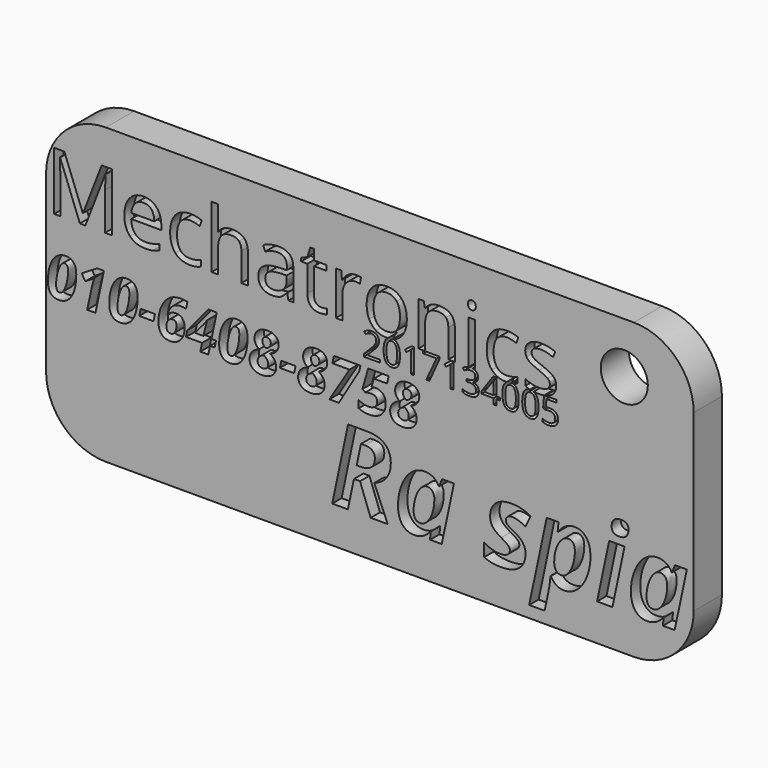
from build123d import *

# Parameters (mm, degrees)
F0_W           = 55
F0_H           = 25
F1_DEPTH       = 3
F2_TEXT_SIZE   = 4.7299554753
F2_TEXT_SIZE_2 = 8.9130162028
F3_DEPTH       = 1
F4_R           = 5.08
F5_R           = 5.08
F6_R           = 5.08
F7_R           = 5.08
F8_R           = 2
F9_DEPTH       = 3


# Not quite as in the source:
# - Text() gives the source's letters only with a copy of the font that has no kerning and outlines rounded to 1/6400 em; it was checked with that copy


with BuildPart() as f1:
    # F0 (on Front) → F1 (new body)
    with BuildSketch(Plane.XZ):
        with Locations((3.4295588825, -2.7567299395)):
            Rectangle(F0_W, F0_H)
    extrude(amount=F1_DEPTH)

    # F2 (on face) → F3 (cut)
    with BuildSketch(Plane.XZ.offset(3)):
        with Locations((-24.0704411175, -4.4084611423)):
            Text('010-6408-8758', F2_TEXT_SIZE, font='Open Sans', font_style=FontStyle.BOLDITALIC, text_align=(TextAlign.LEFT, TextAlign.BOTTOM))
        with Locations((0, -12.1290959666)):
            Text('Ra spia', F2_TEXT_SIZE_2, font='Open Sans', font_style=FontStyle.BOLDITALIC, text_align=(TextAlign.LEFT, TextAlign.BOTTOM))
        with BuildLine():
            Line((-22.8788005036, 6.2329982247), (-21.1996705477, 1.8455941463))
            Line((-21.1996705477, 1.8455941463), (-20.7360140179, 1.8455941463))
            Line((-20.7360140179, 1.8455941463), (-19.0428010365, 6.2264983668))
            Line((-19.0428010365, 6.2264983668), (-19.0157182953, 6.2264983668))
            add(Edge.make_bspline(
                [(-19.0633839198, 5.0348577529), (-19.0633839198, 5.5830124353), (-19.0157182953, 6.2264983668)],
                knots=[0, 0, 0, 1, 1, 1], degree=2))
            Line((-19.0633839198, 5.0348577529), (-19.0633839198, 1.8455941463))
            Line((-19.0633839198, 1.8455941463), (-18.4881464962, 1.8455941463))
            Line((-18.4881464962, 1.8455941463), (-18.4881464962, 6.7952359326))
            Line((-18.4881464962, 6.7952359326), (-19.3482943575, 6.7952359326))
            Line((-19.3482943575, 6.7952359326), (-20.9288431354, 2.7122418655))
            Line((-20.9288431354, 2.7122418655), (-20.9559258766, 2.7122418655))
            Line((-20.9559258766, 2.7122418655), (-22.5234749387, 6.7952359326))
            Line((-22.5234749387, 6.7952359326), (-23.3901226579, 6.7952359326))
            Line((-23.3901226579, 6.7952359326), (-23.3901226579, 1.8455941463))
            Line((-23.3901226579, 1.8455941463), (-22.8582176203, 1.8455941463))
            Line((-22.8582176203, 1.8455941463), (-22.8582176203, 4.9936919863))
            add(Edge.make_bspline(
                [(-22.9058832448, 6.2329982247), (-22.8582176203, 5.7119262836), (-22.8582176203, 4.9936919863)],
                knots=[0, 0, 0, 1, 1, 1], degree=2))
            Line((-22.9058832448, 6.2329982247), (-22.8788005036, 6.2329982247))
        make_face()
        with BuildLine():
            add(Edge.make_bspline(
                [(-15.6477085965, 1.7773456384), (-16.4699406201, 1.7773456384), (-16.9460552109, 2.2789180059)],
                knots=[0, 0, 0, 1, 1, 1], degree=2))
            add(Edge.make_bspline(
                [(-15.0063892843, 1.8336777401), (-15.2718001483, 1.7773456384), (-15.6477085965, 1.7773456384)],
                knots=[0, 0, 0, 1, 1, 1], degree=2))
            add(Edge.make_bspline(
                [(-14.4430682669, 2.0178403805), (-14.7409784203, 1.8900098419), (-15.0063892843, 1.8336777401)],
                knots=[0, 0, 0, 1, 1, 1], degree=2))
            Line((-14.4430682669, 2.0178403805), (-14.4430682669, 2.519412748))
            add(Edge.make_bspline(
                [(-15.6271257132, 2.269168219), (-15.0280554773, 2.269168219), (-14.4430682669, 2.519412748)],
                knots=[0, 0, 0, 1, 1, 1], degree=2))
            add(Edge.make_bspline(
                [(-16.5089397675, 2.6077024844), (-16.1958632789, 2.269168219), (-15.6271257132, 2.269168219)],
                knots=[0, 0, 0, 1, 1, 1], degree=2))
            add(Edge.make_bspline(
                [(-16.8393492104, 3.599472468), (-16.8220162561, 2.9462367497), (-16.5089397675, 2.6077024844)],
                knots=[0, 0, 0, 1, 1, 1], degree=2))
            Line((-16.8393492104, 3.599472468), (-14.2838217485, 3.599472468))
            Line((-14.2838217485, 3.599472468), (-14.2838217485, 3.9547980329))
            add(Edge.make_bspline(
                [(-14.6900628668, 5.1653965656), (-14.2838217485, 4.7066149293), (-14.2838217485, 3.9547980329)],
                knots=[0, 0, 0, 1, 1, 1], degree=2))
            add(Edge.make_bspline(
                [(-15.7928720895, 5.624178202), (-15.0963039852, 5.624178202), (-14.6900628668, 5.1653965656)],
                knots=[0, 0, 0, 1, 1, 1], degree=2))
            add(Edge.make_bspline(
                [(-16.9801794648, 5.0960647481), (-16.538189128, 5.624178202), (-15.7928720895, 5.624178202)],
                knots=[0, 0, 0, 1, 1, 1], degree=2))
            add(Edge.make_bspline(
                [(-17.4221698016, 3.6698875952), (-17.4221698016, 4.5679512942), (-16.9801794648, 5.0960647481)],
                knots=[0, 0, 0, 1, 1, 1], degree=2))
            add(Edge.make_bspline(
                [(-16.9460552109, 2.2789180059), (-17.4221698016, 2.7804903734), (-17.4221698016, 3.6698875952)],
                knots=[0, 0, 0, 1, 1, 1], degree=2))
        make_face()
        with BuildLine():
            add(Edge.make_bspline(
                [(-15.8004552571, 5.1529385047), (-16.2467788324, 5.1529385047), (-16.5127313513, 4.8620698639)],
                knots=[0, 0, 0, 1, 1, 1], degree=2))
            add(Edge.make_bspline(
                [(-15.1228450716, 4.8701946863), (-15.3595482299, 5.1529385047), (-15.8004552571, 5.1529385047)],
                knots=[0, 0, 0, 1, 1, 1], degree=2))
            add(Edge.make_bspline(
                [(-14.8861419133, 4.0566291399), (-14.8861419133, 4.5874508679), (-15.1228450716, 4.8701946863)],
                knots=[0, 0, 0, 1, 1, 1], degree=2))
            Line((-14.8861419133, 4.0566291399), (-16.8263494947, 4.0566291399))
            add(Edge.make_bspline(
                [(-16.5127313513, 4.8620698639), (-16.7786838701, 4.5712012232), (-16.8263494947, 4.0566291399)],
                knots=[0, 0, 0, 1, 1, 1], degree=2))
        make_face(mode=Mode.SUBTRACT)
        with BuildLine():
            add(Edge.make_bspline(
                [(-11.8420417996, 1.7773456384), (-12.6480241785, 1.7773456384), (-13.0900145153, 2.2735014576)],
                knots=[0, 0, 0, 1, 1, 1], degree=2))
            add(Edge.make_bspline(
                [(-10.9049789532, 1.9712580656), (-11.2765541628, 1.7773456384), (-11.8420417996, 1.7773456384)],
                knots=[0, 0, 0, 1, 1, 1], degree=2))
            Line((-10.9049789532, 1.9712580656), (-10.9049789532, 2.4684971945))
            add(Edge.make_bspline(
                [(-11.8561248251, 2.269168219), (-11.3924682953, 2.269168219), (-10.9049789532, 2.4684971945)],
                knots=[0, 0, 0, 1, 1, 1], degree=2))
            add(Edge.make_bspline(
                [(-12.6734819552, 2.6347852256), (-12.3977796496, 2.269168219), (-11.8561248251, 2.269168219)],
                knots=[0, 0, 0, 1, 1, 1], degree=2))
            add(Edge.make_bspline(
                [(-12.9491842609, 3.6839706206), (-12.9491842609, 3.0004022321), (-12.6734819552, 2.6347852256)],
                knots=[0, 0, 0, 1, 1, 1], degree=2))
            add(Edge.make_bspline(
                [(-11.8182089873, 5.1258557635), (-12.9491842609, 5.1258557635), (-12.9491842609, 3.6839706206)],
                knots=[0, 0, 0, 1, 1, 1], degree=2))
            add(Edge.make_bspline(
                [(-11.4293008233, 5.0771068293), (-11.6492126821, 5.1258557635), (-11.8182089873, 5.1258557635)],
                knots=[0, 0, 0, 1, 1, 1], degree=2))
            add(Edge.make_bspline(
                [(-11.023059705, 4.9536095293), (-11.2093889646, 5.028357895), (-11.4293008233, 5.0771068293)],
                knots=[0, 0, 0, 1, 1, 1], degree=2))
            Line((-11.023059705, 4.9536095293), (-10.8508134708, 5.4302657748))
            add(Edge.make_bspline(
                [(-11.2700543049, 5.5662211358), (-11.0024768216, 5.5082640696), (-10.8508134708, 5.4302657748)],
                knots=[0, 0, 0, 1, 1, 1], degree=2))
            add(Edge.make_bspline(
                [(-11.8052092716, 5.624178202), (-11.5376317882, 5.624178202), (-11.2700543049, 5.5662211358)],
                knots=[0, 0, 0, 1, 1, 1], degree=2))
            add(Edge.make_bspline(
                [(-13.0829730025, 5.1161059766), (-12.633941153, 5.624178202), (-11.8052092716, 5.624178202)],
                knots=[0, 0, 0, 1, 1, 1], degree=2))
            add(Edge.make_bspline(
                [(-13.5320048521, 3.6774707627), (-13.5320048521, 4.6080337512), (-13.0829730025, 5.1161059766)],
                knots=[0, 0, 0, 1, 1, 1], degree=2))
            add(Edge.make_bspline(
                [(-13.0900145153, 2.2735014576), (-13.5320048521, 2.7696572769), (-13.5320048521, 3.6774707627)],
                knots=[0, 0, 0, 1, 1, 1], degree=2))
        make_face()
        with BuildLine():
            Line((-7.4849703913, 4.2462083285), (-7.4849703913, 1.8455941463))
            Line((-7.4849703913, 1.8455941463), (-6.9227326835, 1.8455941463))
            Line((-6.9227326835, 1.8455941463), (-6.9227326835, 4.2657079022))
            add(Edge.make_bspline(
                [(-7.2634335681, 5.2932271042), (-6.9227326835, 4.969859174), (-6.9227326835, 4.2657079022)],
                knots=[0, 0, 0, 1, 1, 1], degree=2))
            add(Edge.make_bspline(
                [(-8.2844529123, 5.6165950345), (-7.6041344527, 5.6165950345), (-7.2634335681, 5.2932271042)],
                knots=[0, 0, 0, 1, 1, 1], degree=2))
            add(Edge.make_bspline(
                [(-8.9831876359, 5.4627650643), (-8.6766110052, 5.6165950345), (-8.2844529123, 5.6165950345)],
                knots=[0, 0, 0, 1, 1, 1], degree=2))
            add(Edge.make_bspline(
                [(-9.4555106429, 5.0413576108), (-9.2897642666, 5.3089350941), (-8.9831876359, 5.4627650643)],
                knots=[0, 0, 0, 1, 1, 1], degree=2))
            Line((-9.4555106429, 5.0413576108), (-9.489093242, 5.0413576108))
            add(Edge.make_bspline(
                [(-9.4620105008, 5.519097166), (-9.4620105008, 5.2309367994), (-9.489093242, 5.0413576108)],
                knots=[0, 0, 0, 1, 1, 1], degree=2))
            Line((-9.4620105008, 5.519097166), (-9.4620105008, 7.1137289694))
            Line((-9.4620105008, 7.1137289694), (-10.0242482086, 7.1137289694))
            Line((-10.0242482086, 7.1137289694), (-10.0242482086, 1.8455941463))
            Line((-10.0242482086, 1.8455941463), (-9.4620105008, 1.8455941463))
            Line((-9.4620105008, 1.8455941463), (-9.4620105008, 3.7858017276))
            add(Edge.make_bspline(
                [(-9.192808053, 4.82794561), (-9.4620105008, 4.5094525732), (-9.4620105008, 3.7858017276)],
                knots=[0, 0, 0, 1, 1, 1], degree=2))
            add(Edge.make_bspline(
                [(-8.3386183948, 5.1464386468), (-8.9236056052, 5.1464386468), (-9.192808053, 4.82794561)],
                knots=[0, 0, 0, 1, 1, 1], degree=2))
            add(Edge.make_bspline(
                [(-7.6913408795, 4.9227352043), (-7.8977113676, 5.1464386468), (-8.3386183948, 5.1464386468)],
                knots=[0, 0, 0, 1, 1, 1], degree=2))
            add(Edge.make_bspline(
                [(-7.4849703913, 4.2462083285), (-7.4849703913, 4.6990317618), (-7.6913408795, 4.9227352043)],
                knots=[0, 0, 0, 1, 1, 1], degree=2))
        make_face()
        with BuildLine():
            Line((-3.5991386804, 2.374249255), (-3.4875577865, 1.8455941463))
            Line((-3.4875577865, 1.8455941463), (-3.0704835717, 1.8455941463))
            Line((-3.0704835717, 1.8455941463), (-3.0704835717, 4.3783721056))
            add(Edge.make_bspline(
                [(-3.390601573, 5.3224764647), (-3.0704835717, 5.028357895), (-3.0704835717, 4.3783721056)],
                knots=[0, 0, 0, 1, 1, 1], degree=2))
            add(Edge.make_bspline(
                [(-4.3737050794, 5.6165950345), (-3.7107195742, 5.6165950345), (-3.390601573, 5.3224764647)],
                knots=[0, 0, 0, 1, 1, 1], degree=2))
            add(Edge.make_bspline(
                [(-5.0296490719, 5.5320968818), (-4.7030312127, 5.6165950345), (-4.3737050794, 5.6165950345)],
                knots=[0, 0, 0, 1, 1, 1], degree=2))
            add(Edge.make_bspline(
                [(-5.6303442723, 5.2991853073), (-5.3562669311, 5.4475987292), (-5.0296490719, 5.5320968818)],
                knots=[0, 0, 0, 1, 1, 1], degree=2))
            Line((-5.6303442723, 5.2991853073), (-5.4570147284, 4.8691113766))
            add(Edge.make_bspline(
                [(-4.4083709882, 5.1529385047), (-4.872027518, 5.1529385047), (-5.4570147284, 4.8691113766)],
                knots=[0, 0, 0, 1, 1, 1], degree=2))
            add(Edge.make_bspline(
                [(-3.807134133, 4.9449430521), (-3.9945467023, 5.1529385047), (-4.4083709882, 5.1529385047)],
                knots=[0, 0, 0, 1, 1, 1], degree=2))
            add(Edge.make_bspline(
                [(-3.6197215637, 4.3003738109), (-3.6197215637, 4.7369475995), (-3.807134133, 4.9449430521)],
                knots=[0, 0, 0, 1, 1, 1], degree=2))
            Line((-3.6197215637, 4.3003738109), (-3.6197215637, 4.0696288557))
            Line((-3.6197215637, 4.0696288557), (-4.2491244698, 4.0490459724))
            add(Edge.make_bspline(
                [(-6.0463351775, 2.8714883839), (-6.0463351775, 3.9948804899), (-4.2491244698, 4.0490459724)],
                knots=[0, 0, 0, 1, 1, 1], degree=2))
            add(Edge.make_bspline(
                [(-5.7332586889, 2.0622560761), (-6.0463351775, 2.3471665138), (-6.0463351775, 2.8714883839)],
                knots=[0, 0, 0, 1, 1, 1], degree=2))
            add(Edge.make_bspline(
                [(-4.868777589, 1.7773456384), (-5.4201822004, 1.7773456384), (-5.7332586889, 2.0622560761)],
                knots=[0, 0, 0, 1, 1, 1], degree=2))
            add(Edge.make_bspline(
                [(-4.1792509974, 1.9013845932), (-4.4549533031, 1.7773456384), (-4.868777589, 1.7773456384)],
                knots=[0, 0, 0, 1, 1, 1], degree=2))
            add(Edge.make_bspline(
                [(-3.6262214216, 2.374249255), (-3.9035486918, 2.025423548), (-4.1792509974, 1.9013845932)],
                knots=[0, 0, 0, 1, 1, 1], degree=2))
            Line((-3.6262214216, 2.374249255), (-3.5991386804, 2.374249255))
        make_face()
        with BuildLine():
            add(Edge.make_bspline(
                [(-4.7571966952, 2.2420854778), (-4.2317915154, 2.2420854778), (-3.9322563975, 2.5297041896)],
                knots=[0, 0, 0, 1, 1, 1], degree=2))
            add(Edge.make_bspline(
                [(-5.2728520881, 2.4007903414), (-5.0886894478, 2.2420854778), (-4.7571966952, 2.2420854778)],
                knots=[0, 0, 0, 1, 1, 1], degree=2))
            add(Edge.make_bspline(
                [(-5.4570147284, 2.864988526), (-5.4570147284, 2.559495205), (-5.2728520881, 2.4007903414)],
                knots=[0, 0, 0, 1, 1, 1], degree=2))
            add(Edge.make_bspline(
                [(-5.1612711942, 3.4386009851), (-5.4570147284, 3.25389669), (-5.4570147284, 2.864988526)],
                knots=[0, 0, 0, 1, 1, 1], degree=2))
            add(Edge.make_bspline(
                [(-4.1949589873, 3.6471380926), (-4.8655276601, 3.6233052803), (-5.1612711942, 3.4386009851)],
                knots=[0, 0, 0, 1, 1, 1], degree=2))
            Line((-4.1949589873, 3.6471380926), (-3.6327212795, 3.6698875952))
            Line((-3.6327212795, 3.6698875952), (-3.6327212795, 3.3351449137))
            add(Edge.make_bspline(
                [(-3.9322563975, 2.5297041896), (-3.6327212795, 2.8173229014), (-3.6327212795, 3.3351449137)],
                knots=[0, 0, 0, 1, 1, 1], degree=2))
        make_face(mode=Mode.SUBTRACT)
        with BuildLine():
            add(Edge.make_bspline(
                [(-0.7153683948, 2.2420854778), (-0.5658716632, 2.2420854778), (-0.4272080281, 2.2637516708)],
                knots=[0, 0, 0, 1, 1, 1], degree=2))
            add(Edge.make_bspline(
                [(-1.1519421833, 2.4213732247), (-0.9926956649, 2.2420854778), (-0.7153683948, 2.2420854778)],
                knots=[0, 0, 0, 1, 1, 1], degree=2))
            add(Edge.make_bspline(
                [(-1.3111887017, 2.9354036532), (-1.3111887017, 2.6006609716), (-1.1519421833, 2.4213732247)],
                knots=[0, 0, 0, 1, 1, 1], degree=2))
            Line((-1.3111887017, 2.9354036532), (-1.3111887017, 5.1193559056))
            Line((-1.3111887017, 5.1193559056), (-0.2343789106, 5.1193559056))
            Line((-0.2343789106, 5.1193559056), (-0.2343789106, 5.5559296941))
            Line((-0.2343789106, 5.5559296941), (-1.3111887017, 5.5559296941))
            Line((-1.3111887017, 5.5559296941), (-1.3111887017, 6.4160775554))
            Line((-1.3111887017, 6.4160775554), (-1.6361815964, 6.4160775554))
            Line((-1.6361815964, 6.4160775554), (-1.8723430999, 5.624178202))
            Line((-1.8723430999, 5.624178202), (-2.4042481375, 5.3901833178))
            Line((-2.4042481375, 5.3901833178), (-2.4042481375, 5.1193559056))
            Line((-2.4042481375, 5.1193559056), (-1.8723430999, 5.1193559056))
            Line((-1.8723430999, 5.1193559056), (-1.8723430999, 2.9115708409))
            add(Edge.make_bspline(
                [(-0.7966166184, 1.7773456384), (-1.8723430999, 1.7773456384), (-1.8723430999, 2.9115708409)],
                knots=[0, 0, 0, 1, 1, 1], degree=2))
            add(Edge.make_bspline(
                [(-0.4759569623, 1.8065949989), (-0.6536197448, 1.7773456384), (-0.7966166184, 1.7773456384)],
                knots=[0, 0, 0, 1, 1, 1], degree=2))
            add(Edge.make_bspline(
                [(-0.2072961694, 1.8791767454), (-0.2982941799, 1.8358443594), (-0.4759569623, 1.8065949989)],
                knots=[0, 0, 0, 1, 1, 1], degree=2))
            Line((-0.2072961694, 1.8791767454), (-0.2072961694, 2.3092506761))
            add(Edge.make_bspline(
                [(-0.4272080281, 2.2637516708), (-0.2885443931, 2.2854178638), (-0.2072961694, 2.3092506761)],
                knots=[0, 0, 0, 1, 1, 1], degree=2))
        make_face()
        with BuildLine():
            add(Edge.make_bspline(
                [(2.2269006119, 5.624178202), (2.4738952119, 5.624178202), (2.6699742584, 5.5830124353)],
                knots=[0, 0, 0, 1, 1, 1], degree=2))
            add(Edge.make_bspline(
                [(1.5866646094, 5.4275575007), (1.8780749049, 5.624178202), (2.2269006119, 5.624178202)],
                knots=[0, 0, 0, 1, 1, 1], degree=2))
            add(Edge.make_bspline(
                [(1.0894254805, 4.8691113766), (1.2952543138, 5.2309367994), (1.5866646094, 5.4275575007)],
                knots=[0, 0, 0, 1, 1, 1], degree=2))
            Line((1.0894254805, 4.8691113766), (1.0623427393, 4.8691113766))
            Line((1.0623427393, 4.8691113766), (0.9973441603, 5.5559296941))
            Line((0.9973441603, 5.5559296941), (0.5336876305, 5.5559296941))
            Line((0.5336876305, 5.5559296941), (0.5336876305, 1.8455941463))
            Line((0.5336876305, 1.8455941463), (1.0959253384, 1.8455941463))
            Line((1.0959253384, 1.8455941463), (1.0959253384, 3.8367172811))
            add(Edge.make_bspline(
                [(1.4155016848, 4.7472390411), (1.0959253384, 4.3816220346), (1.0959253384, 3.8367172811)],
                knots=[0, 0, 0, 1, 1, 1], degree=2))
            add(Edge.make_bspline(
                [(2.1857348453, 5.1128560477), (1.7350780313, 5.1128560477), (1.4155016848, 4.7472390411)],
                knots=[0, 0, 0, 1, 1, 1], degree=2))
            add(Edge.make_bspline(
                [(2.5919759636, 5.0619404942), (2.362314318, 5.1128560477), (2.1857348453, 5.1128560477)],
                knots=[0, 0, 0, 1, 1, 1], degree=2))
            Line((2.5919759636, 5.0619404942), (2.6699742584, 5.5830124353))
        make_face()
        with BuildLine():
            add(Edge.make_bspline(
                [(6.5666390658, 3.704553504), (6.5666390658, 2.7967400181), (6.1100240488, 2.2870428283)],
                knots=[0, 0, 0, 1, 1, 1], degree=2))
            add(Edge.make_bspline(
                [(6.1078574295, 5.1058145349), (6.5666390658, 4.5874508679), (6.5666390658, 3.704553504)],
                knots=[0, 0, 0, 1, 1, 1], degree=2))
            add(Edge.make_bspline(
                [(4.8712594651, 5.624178202), (5.6490757931, 5.624178202), (6.1078574295, 5.1058145349)],
                knots=[0, 0, 0, 1, 1, 1], degree=2))
            add(Edge.make_bspline(
                [(3.6113703433, 5.1177309411), (4.0652770863, 5.624178202), (4.8712594651, 5.624178202)],
                knots=[0, 0, 0, 1, 1, 1], degree=2))
            add(Edge.make_bspline(
                [(3.1574636004, 3.704553504), (3.1574636004, 4.6112836802), (3.6113703433, 5.1177309411)],
                knots=[0, 0, 0, 1, 1, 1], degree=2))
            add(Edge.make_bspline(
                [(3.3676256723, 2.6819091953), (3.1574636004, 3.1184829839), (3.1574636004, 3.704553504)],
                knots=[0, 0, 0, 1, 1, 1], degree=2))
            add(Edge.make_bspline(
                [(3.9634459793, 2.0113405226), (3.5777877442, 2.2453354068), (3.3676256723, 2.6819091953)],
                knots=[0, 0, 0, 1, 1, 1], degree=2))
            add(Edge.make_bspline(
                [(4.8474266529, 1.7773456384), (4.3491042143, 1.7773456384), (3.9634459793, 2.0113405226)],
                knots=[0, 0, 0, 1, 1, 1], degree=2))
            add(Edge.make_bspline(
                [(4.955877792, 1.7797225946), (4.9024668541, 1.7773456384), (4.8474266529, 1.7773456384)],
                knots=[0.9317104162, 0.9317104162, 0.9317104162, 1, 1, 1], degree=2))
            add(Edge.make_bspline(
                [(4.955877792, 1.7797225946), (5.0945894967, 1.8607604798), (5.2879334835, 1.8607604798)],
                knots=[0.4479110722, 0.4479110722, 0.4479110722, 1, 1, 1], degree=2))
            add(Edge.make_bspline(
                [(5.2879334835, 1.8607604798), (5.3518272745, 1.8607604798), (5.409976095, 1.8510758715)],
                knots=[0, 0, 0, 0.1868611686, 0.1868611686, 0.1868611686], degree=2))
            add(Edge.make_bspline(
                [(6.1100240488, 2.2870428283), (5.8270758606, 1.9712014937), (5.409976095, 1.8510758715)],
                knots=[0, 0, 0, 0.6196646574, 0.6196646574, 0.6196646574], degree=2))
        make_face()
        with BuildLine():
            add(Edge.make_bspline(
                [(3.7402841916, 3.704553504), (3.7402841916, 2.9928190646), (4.0246529744, 2.6207022001)],
                knots=[0, 0, 0, 1, 1, 1], degree=2))
            add(Edge.make_bspline(
                [(4.0214030455, 4.7840715692), (3.7402841916, 4.4217044916), (3.7402841916, 3.704553504)],
                knots=[0, 0, 0, 1, 1, 1], degree=2))
            add(Edge.make_bspline(
                [(4.8539265107, 5.1464386468), (4.3025218994, 5.1464386468), (4.0214030455, 4.7840715692)],
                knots=[0, 0, 0, 1, 1, 1], degree=2))
            add(Edge.make_bspline(
                [(5.698908037, 4.7791966758), (5.4129142896, 5.1464386468), (4.8539265107, 5.1464386468)],
                knots=[0, 0, 0, 1, 1, 1], degree=2))
            add(Edge.make_bspline(
                [(5.9849017843, 3.704553504), (5.9849017843, 4.4119547048), (5.698908037, 4.7791966758)],
                knots=[0, 0, 0, 1, 1, 1], degree=2))
            add(Edge.make_bspline(
                [(5.698908037, 2.6190772357), (5.9849017843, 2.9895691356), (5.9849017843, 3.704553504)],
                knots=[0, 0, 0, 1, 1, 1], degree=2))
            add(Edge.make_bspline(
                [(4.8604263686, 2.2485853357), (5.4129142896, 2.2485853357), (5.698908037, 2.6190772357)],
                knots=[0, 0, 0, 1, 1, 1], degree=2))
            add(Edge.make_bspline(
                [(4.0246529744, 2.6207022001), (4.3090217573, 2.2485853357), (4.8604263686, 2.2485853357)],
                knots=[0, 0, 0, 1, 1, 1], degree=2))
        make_face(mode=Mode.SUBTRACT)
        with BuildLine():
            add(Edge.make_bspline(
                [(5.409976095, 1.8510758715), (5.6630145634, 1.8089326533), (5.8072655083, 1.5834004116)],
                knots=[0.1868611686, 0.1868611686, 0.1868611686, 1, 1, 1], degree=2))
            add(Edge.make_bspline(
                [(5.409976095, 1.8510758715), (5.1999363399, 1.7905839741), (4.955877792, 1.7797225946)],
                knots=[0.6196646574, 0.6196646574, 0.6196646574, 0.9317104162, 0.9317104162, 0.9317104162], degree=2))
            add(Edge.make_bspline(
                [(4.7667631152, 1.5948900582), (4.8433406531, 1.7139763638), (4.955877792, 1.7797225946)],
                knots=[0, 0, 0, 0.4479110722, 0.4479110722, 0.4479110722], degree=2))
            add(Edge.make_bspline(
                [(4.5957971743, 0.7807337024), (4.5957971743, 1.3290196366), (4.7667631152, 1.5948900582)],
                knots=[0, 0, 0, 1, 1, 1], degree=2))
            add(Edge.make_bspline(
                [(4.7725079385, -0.0260692796), (4.5957971743, 0.2489928593), (4.5957971743, 0.7807337024)],
                knots=[0, 0, 0, 1, 1, 1], degree=2))
            add(Edge.make_bspline(
                [(5.2879334835, -0.3011314184), (4.9492187027, -0.3011314184), (4.7725079385, -0.0260692796)],
                knots=[0, 0, 0, 1, 1, 1], degree=2))
            add(Edge.make_bspline(
                [(5.8130103316, -0.0325034816), (5.6413550119, -0.3011314184), (5.2879334835, -0.3011314184)],
                knots=[0, 0, 0, 1, 1, 1], degree=2))
            add(Edge.make_bspline(
                [(5.9846656513, 0.7807337024), (5.9846656513, 0.2361244551), (5.8130103316, -0.0325034816)],
                knots=[0, 0, 0, 1, 1, 1], degree=2))
            add(Edge.make_bspline(
                [(5.8072655083, 1.5834004116), (5.9846656513, 1.3060403435), (5.9846656513, 0.7807337024)],
                knots=[0, 0, 0, 1, 1, 1], degree=2))
        make_face()
        with BuildLine():
            add(Edge.make_bspline(
                [(4.8370797522, 0.7807337024), (4.8370797522, 0.3225265973), (4.944852637, 0.1134150298)],
                knots=[0, 0, 0, 1, 1, 1], degree=2))
            add(Edge.make_bspline(
                [(4.944852637, 1.4464438245), (4.8370797522, 1.2389408075), (4.8370797522, 0.7807337024)],
                knots=[0, 0, 0, 1, 1, 1], degree=2))
            add(Edge.make_bspline(
                [(5.2879334835, 1.6539468415), (5.0526255218, 1.6539468415), (4.944852637, 1.4464438245)],
                knots=[0, 0, 0, 1, 1, 1], degree=2))
            add(Edge.make_bspline(
                [(5.6333122593, 1.4434565164), (5.5264585462, 1.6539468415), (5.2879334835, 1.6539468415)],
                knots=[0, 0, 0, 1, 1, 1], degree=2))
            add(Edge.make_bspline(
                [(5.7401659724, 0.7807337024), (5.7401659724, 1.2329661913), (5.6333122593, 1.4434565164)],
                knots=[0, 0, 0, 1, 1, 1], degree=2))
            add(Edge.make_bspline(
                [(5.6333122593, 0.1161725449), (5.7401659724, 0.3280416277), (5.7401659724, 0.7807337024)],
                knots=[0, 0, 0, 1, 1, 1], degree=2))
            add(Edge.make_bspline(
                [(5.2879334835, -0.0956965378), (5.5264585462, -0.0956965378), (5.6333122593, 0.1161725449)],
                knots=[0, 0, 0, 1, 1, 1], degree=2))
            add(Edge.make_bspline(
                [(4.944852637, 0.1134150298), (5.0526255218, -0.0956965378), (5.2879334835, -0.0956965378)],
                knots=[0, 0, 0, 1, 1, 1], degree=2))
        make_face(mode=Mode.SUBTRACT)
        with BuildLine():
            add(Edge.make_bspline(
                [(5.409976095, 1.8510758715), (5.1999363399, 1.7905839741), (4.955877792, 1.7797225946)],
                knots=[0.6196646574, 0.6196646574, 0.6196646574, 0.9317104162, 0.9317104162, 0.9317104162], degree=2))
            add(Edge.make_bspline(
                [(5.2879334835, 1.8607604798), (5.3518272745, 1.8607604798), (5.409976095, 1.8510758715)],
                knots=[0, 0, 0, 0.1868611686, 0.1868611686, 0.1868611686], degree=2))
            add(Edge.make_bspline(
                [(4.955877792, 1.7797225946), (5.0945894967, 1.8607604798), (5.2879334835, 1.8607604798)],
                knots=[0.4479110722, 0.4479110722, 0.4479110722, 1, 1, 1], degree=2))
        make_face()
        with BuildLine():
            Line((10.0917286637, 4.2462083285), (10.0917286637, 1.8455941463))
            Line((10.0917286637, 1.8455941463), (10.6539663715, 1.8455941463))
            Line((10.6539663715, 1.8455941463), (10.6539663715, 4.2657079022))
            add(Edge.make_bspline(
                [(10.3154321062, 5.3008102718), (10.6539663715, 4.9774423415), (10.6539663715, 4.2657079022)],
                knots=[0, 0, 0, 1, 1, 1], degree=2))
            add(Edge.make_bspline(
                [(9.3063291681, 5.624178202), (9.9768978409, 5.624178202), (10.3154321062, 5.3008102718)],
                knots=[0, 0, 0, 1, 1, 1], degree=2))
            add(Edge.make_bspline(
                [(8.6124693379, 5.473056506), (8.923920862, 5.624178202), (9.3063291681, 5.624178202)],
                knots=[0, 0, 0, 1, 1, 1], degree=2))
            add(Edge.make_bspline(
                [(8.12768827, 5.0478574687), (8.3010178139, 5.3219348099), (8.6124693379, 5.473056506)],
                knots=[0, 0, 0, 1, 1, 1], degree=2))
            Line((8.12768827, 5.0478574687), (8.1006055288, 5.0478574687))
            Line((8.1006055288, 5.0478574687), (8.0096075183, 5.5559296941))
            Line((8.0096075183, 5.5559296941), (7.5524508464, 5.5559296941))
            Line((7.5524508464, 5.5559296941), (7.5524508464, 1.8455941463))
            Line((7.5524508464, 1.8455941463), (8.1146885542, 1.8455941463))
            Line((8.1146885542, 1.8455941463), (8.1146885542, 3.7923015855))
            add(Edge.make_bspline(
                [(8.3855159665, 4.8317371938), (8.1146885542, 4.5170357407), (8.1146885542, 3.7923015855)],
                knots=[0, 0, 0, 1, 1, 1], degree=2))
            add(Edge.make_bspline(
                [(9.2380806602, 5.1464386468), (8.6563433787, 5.1464386468), (8.3855159665, 4.8317371938)],
                knots=[0, 0, 0, 1, 1, 1], degree=2))
            add(Edge.make_bspline(
                [(9.8853581755, 4.9227352043), (9.6789876874, 5.1464386468), (9.2380806602, 5.1464386468)],
                knots=[0, 0, 0, 1, 1, 1], degree=2))
            add(Edge.make_bspline(
                [(10.0917286637, 4.2462083285), (10.0917286637, 4.6990317618), (9.8853581755, 4.9227352043)],
                knots=[0, 0, 0, 1, 1, 1], degree=2))
        make_face()
        with BuildLine():
            Line((12.1428235687, 1.8455941463), (12.3699288555, 1.8455941463))
            Line((12.3699288555, 1.8455941463), (12.3699288555, 5.5559296941))
            Line((12.3699288555, 5.5559296941), (11.8076911477, 5.5559296941))
            Line((11.8076911477, 5.5559296941), (11.8076911477, 1.8455941463))
            Line((11.8076911477, 1.8455941463), (11.8100027821, 1.8455941463))
            add(Edge.make_bspline(
                [(11.8100027821, 1.8455941463), (11.8910256631, 1.8575433787), (11.9758269575, 1.8575433787)],
                knots=[0.5466418669, 0.5466418669, 0.5466418669, 1, 1, 1], degree=2))
            add(Edge.make_bspline(
                [(11.9758269575, 1.8575433787), (12.0651331002, 1.8575433787), (12.1428235687, 1.8455941463)],
                knots=[0, 0, 0, 0.2922086215, 0.2922086215, 0.2922086215], degree=2))
        make_face()
        with BuildLine():
            add(Edge.make_bspline(
                [(12.1428235687, 1.8455941463), (12.3310063933, 1.816650566), (12.4510387395, 1.7175994835)],
                knots=[0.2922086215, 0.2922086215, 0.2922086215, 1, 1, 1], degree=2))
            Line((12.1428235687, 1.8455941463), (11.8100027821, 1.8455941463))
            add(Edge.make_bspline(
                [(11.6201074998, 1.7994057671), (11.7123084965, 1.8311862196), (11.8100027821, 1.8455941463)],
                knots=[0, 0, 0, 0.5466418669, 0.5466418669, 0.5466418669], degree=2))
            add(Edge.make_bspline(
                [(11.3222958607, 1.6392400939), (11.4514394882, 1.7412681555), (11.6201074998, 1.7994057671)],
                knots=[0, 0, 0, 1, 1, 1], degree=2))
            Line((11.3222958607, 1.6392400939), (11.4427073568, 1.478385042))
            add(Edge.make_bspline(
                [(11.7214461825, 1.6164905937), (11.5994261359, 1.5790343459), (11.4427073568, 1.478385042)],
                knots=[0, 0, 0, 1, 1, 1], degree=2))
            add(Edge.make_bspline(
                [(11.9813419878, 1.6539468415), (11.843466229, 1.6539468415), (11.7214461825, 1.6164905937)],
                knots=[0, 0, 0, 1, 1, 1], degree=2))
            add(Edge.make_bspline(
                [(12.2678937732, 1.5661659418), (12.1624188178, 1.6539468415), (11.9813419878, 1.6539468415)],
                knots=[0, 0, 0, 1, 1, 1], degree=2))
            add(Edge.make_bspline(
                [(12.3733687287, 1.3248833638), (12.3733687287, 1.478385042), (12.2678937732, 1.5661659418)],
                knots=[0, 0, 0, 1, 1, 1], degree=2))
            add(Edge.make_bspline(
                [(12.2297481466, 1.0238546238), (12.3733687287, 1.1323168874), (12.3733687287, 1.3248833638)],
                knots=[0, 0, 0, 1, 1, 1], degree=2))
            add(Edge.make_bspline(
                [(11.8407087139, 0.9153923602), (12.0861275645, 0.9153923602), (12.2297481466, 1.0238546238)],
                knots=[0, 0, 0, 1, 1, 1], degree=2))
            Line((11.8407087139, 0.9153923602), (11.6311375605, 0.9153923602))
            Line((11.6311375605, 0.9153923602), (11.6311375605, 0.7104170654))
            Line((11.6311375605, 0.7104170654), (11.8379511987, 0.7104170654))
            add(Edge.make_bspline(
                [(12.4381703354, 0.3280416277), (12.4381703354, 0.7104170654), (11.8379511987, 0.7104170654)],
                knots=[0, 0, 0, 1, 1, 1], degree=2))
            add(Edge.make_bspline(
                [(11.8940206739, -0.0984540529), (12.4381703354, -0.0984540529), (12.4381703354, 0.3280416277)],
                knots=[0, 0, 0, 1, 1, 1], degree=2))
            add(Edge.make_bspline(
                [(11.6017240653, -0.0632957344), (11.7561449151, -0.0984540529), (11.8940206739, -0.0984540529)],
                knots=[0, 0, 0, 1, 1, 1], degree=2))
            add(Edge.make_bspline(
                [(11.3108062142, 0.0394217059), (11.4473032154, -0.0281374159), (11.6017240653, -0.0632957344)],
                knots=[0, 0, 0, 1, 1, 1], degree=2))
            Line((11.3108062142, 0.0394217059), (11.3108062142, -0.1876137103))
            add(Edge.make_bspline(
                [(11.5798937368, -0.2758541959), (11.4413285992, -0.2505769735), (11.3108062142, -0.1876137103)],
                knots=[0, 0, 0, 1, 1, 1], degree=2))
            add(Edge.make_bspline(
                [(11.8852885425, -0.3011314184), (11.7184588744, -0.3011314184), (11.5798937368, -0.2758541959)],
                knots=[0, 0, 0, 1, 1, 1], degree=2))
            add(Edge.make_bspline(
                [(12.4767755478, -0.1393571947), (12.268583152, -0.3011314184), (11.8852885425, -0.3011314184)],
                knots=[0, 0, 0, 1, 1, 1], degree=2))
            add(Edge.make_bspline(
                [(12.6849679436, 0.3225265973), (12.6849679436, 0.022417029), (12.4767755478, -0.1393571947)],
                knots=[0, 0, 0, 1, 1, 1], degree=2))
            add(Edge.make_bspline(
                [(12.5629478971, 0.661471171), (12.6849679436, 0.5320977507), (12.6849679436, 0.3225265973)],
                knots=[0, 0, 0, 1, 1, 1], degree=2))
            add(Edge.make_bspline(
                [(12.1881556261, 0.8220964301), (12.4409278505, 0.7908445914), (12.5629478971, 0.661471171)],
                knots=[0, 0, 0, 1, 1, 1], degree=2))
            Line((12.1881556261, 0.8220964301), (12.1881556261, 0.8335860766))
            add(Edge.make_bspline(
                [(12.5077975936, 1.0045520175), (12.3949692643, 0.8767871477), (12.1881556261, 0.8335860766)],
                knots=[0, 0, 0, 1, 1, 1], degree=2))
            add(Edge.make_bspline(
                [(12.6206259229, 1.3336154952), (12.6206259229, 1.1323168874), (12.5077975936, 1.0045520175)],
                knots=[0, 0, 0, 1, 1, 1], degree=2))
            add(Edge.make_bspline(
                [(12.4510387395, 1.7175994835), (12.6206259229, 1.5776555883), (12.6206259229, 1.3336154952)],
                knots=[0, 0, 0, 1, 1, 1], degree=2))
        make_face()
        with BuildLine():
            Line((11.8100027821, 1.8455941463), (12.1428235687, 1.8455941463))
            add(Edge.make_bspline(
                [(11.9758269575, 1.8575433787), (12.0651331002, 1.8575433787), (12.1428235687, 1.8455941463)],
                knots=[0, 0, 0, 0.2922086215, 0.2922086215, 0.2922086215], degree=2))
            add(Edge.make_bspline(
                [(11.8100027821, 1.8455941463), (11.8910256631, 1.8575433787), (11.9758269575, 1.8575433787)],
                knots=[0.5466418669, 0.5466418669, 0.5466418669, 1, 1, 1], degree=2))
        make_face()
        with BuildLine():
            add(Edge.make_bspline(
                [(11.7600255231, 6.5612410484), (11.7600255231, 6.7540701659), (11.8548151174, 6.8439848668)],
                knots=[0, 0, 0, 1, 1, 1], degree=2))
            add(Edge.make_bspline(
                [(11.8548151174, 6.27849723), (11.7600255231, 6.3716618598), (11.7600255231, 6.5612410484)],
                knots=[0, 0, 0, 1, 1, 1], degree=2))
            add(Edge.make_bspline(
                [(12.0926015854, 6.1853326002), (11.9496047117, 6.1853326002), (11.8548151174, 6.27849723)],
                knots=[0, 0, 0, 1, 1, 1], degree=2))
            add(Edge.make_bspline(
                [(12.3260548147, 6.27849723), (12.2280152915, 6.1853326002), (12.0926015854, 6.1853326002)],
                knots=[0, 0, 0, 1, 1, 1], degree=2))
            add(Edge.make_bspline(
                [(12.4240943379, 6.5612410484), (12.4240943379, 6.3716618598), (12.3260548147, 6.27849723)],
                knots=[0, 0, 0, 1, 1, 1], degree=2))
            add(Edge.make_bspline(
                [(12.3260548147, 6.8423599023), (12.4240943379, 6.750820237), (12.4240943379, 6.5612410484)],
                knots=[0, 0, 0, 1, 1, 1], degree=2))
            add(Edge.make_bspline(
                [(12.0926015854, 6.9338995676), (12.2280152915, 6.9338995676), (12.3260548147, 6.8423599023)],
                knots=[0, 0, 0, 1, 1, 1], degree=2))
            add(Edge.make_bspline(
                [(11.8548151174, 6.8439848668), (11.9496047117, 6.9338995676), (12.0926015854, 6.9338995676)],
                knots=[0, 0, 0, 1, 1, 1], degree=2))
        make_face()
        with BuildLine():
            add(Edge.make_bspline(
                [(15.5847922817, 1.8307613597), (15.3414141909, 1.7773456384), (15.0446203789, 1.7773456384)],
                knots=[0.4751541983, 0.4751541983, 0.4751541983, 1, 1, 1], degree=2))
            add(Edge.make_bspline(
                [(15.0446203789, 1.7773456384), (15.0431101099, 1.7773456384), (15.041601119, 1.7773473805)],
                knots=[0, 0, 0, 0.0018738238, 0.0018738238, 0.0018738238], degree=2))
            add(Edge.make_bspline(
                [(14.8565111449, 1.5948900582), (14.9317154144, 1.7118407837), (15.041601119, 1.7773473805)],
                knots=[0, 0, 0, 0.4398786629, 0.4398786629, 0.4398786629], degree=2))
            add(Edge.make_bspline(
                [(14.685545204, 0.7807337024), (14.685545204, 1.3290196366), (14.8565111449, 1.5948900582)],
                knots=[0, 0, 0, 1, 1, 1], degree=2))
            add(Edge.make_bspline(
                [(14.8622559682, -0.0260692796), (14.685545204, 0.2489928593), (14.685545204, 0.7807337024)],
                knots=[0, 0, 0, 1, 1, 1], degree=2))
            add(Edge.make_bspline(
                [(15.3776815132, -0.3011314184), (15.0389667324, -0.3011314184), (14.8622559682, -0.0260692796)],
                knots=[0, 0, 0, 1, 1, 1], degree=2))
            add(Edge.make_bspline(
                [(15.9027583613, -0.0325034816), (15.7311030416, -0.3011314184), (15.3776815132, -0.3011314184)],
                knots=[0, 0, 0, 1, 1, 1], degree=2))
            add(Edge.make_bspline(
                [(16.0744136811, 0.7807337024), (16.0744136811, 0.2361244551), (15.9027583613, -0.0325034816)],
                knots=[0, 0, 0, 1, 1, 1], degree=2))
            add(Edge.make_bspline(
                [(15.8970135381, 1.5834004116), (16.0744136811, 1.3060403435), (16.0744136811, 0.7807337024)],
                knots=[0, 0, 0, 1, 1, 1], degree=2))
            add(Edge.make_bspline(
                [(15.5847922817, 1.8307613597), (15.7779560591, 1.7695433872), (15.8970135381, 1.5834004116)],
                knots=[0.3288760822, 0.3288760822, 0.3288760822, 1, 1, 1], degree=2))
        make_face()
        with BuildLine():
            add(Edge.make_bspline(
                [(14.9268277819, 0.7807337024), (14.9268277819, 0.3225265973), (15.0346006667, 0.1134150298)],
                knots=[0, 0, 0, 1, 1, 1], degree=2))
            add(Edge.make_bspline(
                [(15.0346006667, 1.4464438245), (14.9268277819, 1.2389408075), (14.9268277819, 0.7807337024)],
                knots=[0, 0, 0, 1, 1, 1], degree=2))
            add(Edge.make_bspline(
                [(15.3776815132, 1.6539468415), (15.1423735515, 1.6539468415), (15.0346006667, 1.4464438245)],
                knots=[0, 0, 0, 1, 1, 1], degree=2))
            add(Edge.make_bspline(
                [(15.723060289, 1.4434565164), (15.6162065759, 1.6539468415), (15.3776815132, 1.6539468415)],
                knots=[0, 0, 0, 1, 1, 1], degree=2))
            add(Edge.make_bspline(
                [(15.8299140021, 0.7807337024), (15.8299140021, 1.2329661913), (15.723060289, 1.4434565164)],
                knots=[0, 0, 0, 1, 1, 1], degree=2))
            add(Edge.make_bspline(
                [(15.723060289, 0.1161725449), (15.8299140021, 0.3280416277), (15.8299140021, 0.7807337024)],
                knots=[0, 0, 0, 1, 1, 1], degree=2))
            add(Edge.make_bspline(
                [(15.3776815132, -0.0956965378), (15.6162065759, -0.0956965378), (15.723060289, 0.1161725449)],
                knots=[0, 0, 0, 1, 1, 1], degree=2))
            add(Edge.make_bspline(
                [(15.0346006667, 0.1134150298), (15.1423735515, -0.0956965378), (15.3776815132, -0.0956965378)],
                knots=[0, 0, 0, 1, 1, 1], degree=2))
        make_face(mode=Mode.SUBTRACT)
        with BuildLine():
            add(Edge.make_bspline(
                [(15.0446203789, 1.7773456384), (15.0431101099, 1.7773456384), (15.041601119, 1.7773473805)],
                knots=[0, 0, 0, 0.0018738238, 0.0018738238, 0.0018738238], degree=2))
            add(Edge.make_bspline(
                [(15.5847922817, 1.8307613597), (15.3414141909, 1.7773456384), (15.0446203789, 1.7773456384)],
                knots=[0.4751541983, 0.4751541983, 0.4751541983, 1, 1, 1], degree=2))
            add(Edge.make_bspline(
                [(15.3776815132, 1.8607604798), (15.4901347309, 1.8607604798), (15.5847922817, 1.8307613597)],
                knots=[0, 0, 0, 0.3288760822, 0.3288760822, 0.3288760822], degree=2))
            add(Edge.make_bspline(
                [(15.041601119, 1.7773473805), (15.1815245411, 1.8607604798), (15.3776815132, 1.8607604798)],
                knots=[0.4398786629, 0.4398786629, 0.4398786629, 1, 1, 1], degree=2))
        make_face()
        with BuildLine():
            add(Edge.make_bspline(
                [(15.041601119, 1.7773473805), (14.237809788, 1.778275347), (13.7966476632, 2.2735014576)],
                knots=[0.0018738238, 0.0018738238, 0.0018738238, 1, 1, 1], degree=2))
            add(Edge.make_bspline(
                [(15.041601119, 1.7773473805), (15.1815245411, 1.8607604798), (15.3776815132, 1.8607604798)],
                knots=[0.4398786629, 0.4398786629, 0.4398786629, 1, 1, 1], degree=2))
            add(Edge.make_bspline(
                [(15.3776815132, 1.8607604798), (15.4901347309, 1.8607604798), (15.5847922817, 1.8307613597)],
                knots=[0, 0, 0, 0.3288760822, 0.3288760822, 0.3288760822], degree=2))
            add(Edge.make_bspline(
                [(15.9816832253, 1.9712580656), (15.8051277044, 1.8791197617), (15.5847922817, 1.8307613597)],
                knots=[0, 0, 0, 0.4751541983, 0.4751541983, 0.4751541983], degree=2))
            Line((15.9816832253, 1.9712580656), (15.9816832253, 2.4684971945))
            add(Edge.make_bspline(
                [(15.0305373534, 2.269168219), (15.4941938832, 2.269168219), (15.9816832253, 2.4684971945)],
                knots=[0, 0, 0, 1, 1, 1], degree=2))
            add(Edge.make_bspline(
                [(14.2131802233, 2.6347852256), (14.4888825289, 2.269168219), (15.0305373534, 2.269168219)],
                knots=[0, 0, 0, 1, 1, 1], degree=2))
            add(Edge.make_bspline(
                [(13.9374779176, 3.6839706206), (13.9374779176, 3.0004022321), (14.2131802233, 2.6347852256)],
                knots=[0, 0, 0, 1, 1, 1], degree=2))
            add(Edge.make_bspline(
                [(15.0684531911, 5.1258557635), (13.9374779176, 5.1258557635), (13.9374779176, 3.6839706206)],
                knots=[0, 0, 0, 1, 1, 1], degree=2))
            add(Edge.make_bspline(
                [(15.4573613551, 5.0771068293), (15.2374494964, 5.1258557635), (15.0684531911, 5.1258557635)],
                knots=[0, 0, 0, 1, 1, 1], degree=2))
            add(Edge.make_bspline(
                [(15.8636024735, 4.9536095293), (15.6772732139, 5.028357895), (15.4573613551, 5.0771068293)],
                knots=[0, 0, 0, 1, 1, 1], degree=2))
            Line((15.8636024735, 4.9536095293), (16.0358487077, 5.4302657748))
            add(Edge.make_bspline(
                [(15.6166078735, 5.5662211358), (15.8841853568, 5.5082640696), (16.0358487077, 5.4302657748)],
                knots=[0, 0, 0, 1, 1, 1], degree=2))
            add(Edge.make_bspline(
                [(15.0814529069, 5.624178202), (15.3490303902, 5.624178202), (15.6166078735, 5.5662211358)],
                knots=[0, 0, 0, 1, 1, 1], degree=2))
            add(Edge.make_bspline(
                [(13.8036891759, 5.1161059766), (14.2527210255, 5.624178202), (15.0814529069, 5.624178202)],
                knots=[0, 0, 0, 1, 1, 1], degree=2))
            add(Edge.make_bspline(
                [(13.3546573264, 3.6774707627), (13.3546573264, 4.6080337512), (13.8036891759, 5.1161059766)],
                knots=[0, 0, 0, 1, 1, 1], degree=2))
            add(Edge.make_bspline(
                [(13.7966476632, 2.2735014576), (13.3546573264, 2.7696572769), (13.3546573264, 3.6774707627)],
                knots=[0, 0, 0, 1, 1, 1], degree=2))
        make_face()
        with BuildLine():
            add(Edge.make_bspline(
                [(19.2554449845, 2.8574053585), (19.2554449845, 2.3395833462), (18.8697867495, 2.0584644923)],
                knots=[0, 0, 0, 1, 1, 1], degree=2))
            add(Edge.make_bspline(
                [(19.0236167196, 3.4705586198), (19.2554449845, 3.2268139488), (19.2554449845, 2.8574053585)],
                knots=[0, 0, 0, 1, 1, 1], degree=2))
            add(Edge.make_bspline(
                [(18.1320528785, 3.9547980329), (18.7917884548, 3.7143032908), (19.0236167196, 3.4705586198)],
                knots=[0, 0, 0, 1, 1, 1], degree=2))
            add(Edge.make_bspline(
                [(17.4820670891, 4.2294170289), (17.6510633944, 4.1346274346), (18.1320528785, 3.9547980329)],
                knots=[0, 0, 0, 1, 1, 1], degree=2))
            add(Edge.make_bspline(
                [(17.2366974536, 4.4287460043), (17.3130707839, 4.3242066232), (17.4820670891, 4.2294170289)],
                knots=[0, 0, 0, 1, 1, 1], degree=2))
            add(Edge.make_bspline(
                [(17.1603241234, 4.682782117), (17.1603241234, 4.5332853855), (17.2366974536, 4.4287460043)],
                knots=[0, 0, 0, 1, 1, 1], degree=2))
            add(Edge.make_bspline(
                [(17.3634446826, 5.0278162402), (17.1603241234, 4.9026939758), (17.1603241234, 4.682782117)],
                knots=[0, 0, 0, 1, 1, 1], degree=2))
            add(Edge.make_bspline(
                [(17.9663065022, 5.1529385047), (17.5665652417, 5.1529385047), (17.3634446826, 5.0278162402)],
                knots=[0, 0, 0, 1, 1, 1], degree=2))
            add(Edge.make_bspline(
                [(18.9781177144, 4.9232768591), (18.4202132451, 5.1529385047), (17.9663065022, 5.1529385047)],
                knots=[0, 0, 0, 1, 1, 1], degree=2))
            Line((18.9781177144, 4.9232768591), (19.1785299994, 5.380433531))
            add(Edge.make_bspline(
                [(18.0063889592, 5.624178202), (18.6054591951, 5.624178202), (19.1785299994, 5.380433531)],
                knots=[0, 0, 0, 1, 1, 1], degree=2))
            add(Edge.make_bspline(
                [(16.9945777471, 5.3614756121), (17.3639863374, 5.624178202), (18.0063889592, 5.624178202)],
                knots=[0, 0, 0, 1, 1, 1], degree=2))
            add(Edge.make_bspline(
                [(16.6251691568, 4.6448662793), (16.6251691568, 5.0987730222), (16.9945777471, 5.3614756121)],
                knots=[0, 0, 0, 1, 1, 1], degree=2))
            add(Edge.make_bspline(
                [(16.7318751572, 4.2088341456), (16.6251691568, 4.3913718214), (16.6251691568, 4.6448662793)],
                knots=[0, 0, 0, 1, 1, 1], degree=2))
            add(Edge.make_bspline(
                [(17.0568680519, 3.8822162864), (16.8385811576, 4.0262964697), (16.7318751572, 4.2088341456)],
                knots=[0, 0, 0, 1, 1, 1], degree=2))
            add(Edge.make_bspline(
                [(17.7929769584, 3.5453069856), (17.2751549462, 3.7381361031), (17.0568680519, 3.8822162864)],
                knots=[0, 0, 0, 1, 1, 1], degree=2))
            add(Edge.make_bspline(
                [(18.5263775908, 3.1813149435), (18.3389650215, 3.3351449137), (17.7929769584, 3.5453069856)],
                knots=[0, 0, 0, 1, 1, 1], degree=2))
            add(Edge.make_bspline(
                [(18.71379016, 2.8108230435), (18.71379016, 3.0274849733), (18.5263775908, 3.1813149435)],
                knots=[0, 0, 0, 1, 1, 1], degree=2))
            add(Edge.make_bspline(
                [(18.4770870017, 2.3823740774), (18.71379016, 2.5226626769), (18.71379016, 2.8108230435)],
                knots=[0, 0, 0, 1, 1, 1], degree=2))
            add(Edge.make_bspline(
                [(17.8005601259, 2.2420854778), (18.2403838434, 2.2420854778), (18.4770870017, 2.3823740774)],
                knots=[0, 0, 0, 1, 1, 1], degree=2))
            add(Edge.make_bspline(
                [(17.2096147124, 2.3195421177), (17.5156496882, 2.2420854778), (17.8005601259, 2.2420854778)],
                knots=[0, 0, 0, 1, 1, 1], degree=2))
            add(Edge.make_bspline(
                [(16.6360022532, 2.5324124638), (16.9035797366, 2.3969987576), (17.2096147124, 2.3195421177)],
                knots=[0, 0, 0, 1, 1, 1], degree=2))
            Line((16.6360022532, 2.5324124638), (16.6360022532, 2.0113405226))
            add(Edge.make_bspline(
                [(17.0240813698, 1.8600701365), (16.8033336698, 1.9164754675), (16.6360022532, 2.0113405226)],
                knots=[0.5945849184, 0.5945849184, 0.5945849184, 1, 1, 1], degree=2))
            add(Edge.make_bspline(
                [(17.0240813698, 1.8600701365), (17.0414610773, 1.8607604798), (17.0593061848, 1.8607604798)],
                knots=[0.9490437411, 0.9490437411, 0.9490437411, 1, 1, 1], degree=2))
            add(Edge.make_bspline(
                [(17.0593061848, 1.8607604798), (17.2161332135, 1.8607604798), (17.3383493876, 1.8024150866)],
                knots=[0, 0, 0, 0.4586499154, 0.4586499154, 0.4586499154], degree=2))
            add(Edge.make_bspline(
                [(17.7864771005, 1.7773456384), (17.545003905, 1.7773456384), (17.3383493876, 1.8024150866)],
                knots=[0, 0, 0, 0.3273174853, 0.3273174853, 0.3273174853], degree=2))
            add(Edge.make_bspline(
                [(18.2210349688, 1.8092358332), (18.0214523277, 1.7773456384), (17.7864771005, 1.7773456384)],
                knots=[0.6631910686, 0.6631910686, 0.6631910686, 1, 1, 1], degree=2))
            Line((18.2210349688, 1.8092358332), (18.2225180033, 1.8276702976))
            Line((18.2225180033, 1.8276702976), (18.3209813571, 1.8276702976))
            add(Edge.make_bspline(
                [(18.8697867495, 2.0584644923), (18.6473014189, 1.8962876853), (18.3209813571, 1.8276702976)],
                knots=[0, 0, 0, 0.5768976528, 0.5768976528, 0.5768976528], degree=2))
        make_face()
        with BuildLine():
            Line((19.2666970834, 1.8276702976), (18.3209813571, 1.8276702976))
            add(Edge.make_bspline(
                [(18.3209813571, 1.8276702976), (18.2721697999, 1.8174063821), (18.2210349688, 1.8092358332)],
                knots=[0.5768976528, 0.5768976528, 0.5768976528, 0.6631910686, 0.6631910686, 0.6631910686], degree=2))
            Line((18.2210349688, 1.8092358332), (18.1434692349, 0.8450757232))
            Line((18.1434692349, 0.8450757232), (18.267097832, 0.7660269548))
            add(Edge.make_bspline(
                [(18.632009007, 0.8078492683), (18.4955120058, 0.8078492683), (18.267097832, 0.7660269548)],
                knots=[0, 0, 0, 1, 1, 1], degree=2))
            add(Edge.make_bspline(
                [(19.1701840522, 0.3684851836), (19.1701840522, 0.8078492683), (18.632009007, 0.8078492683)],
                knots=[0, 0, 0, 1, 1, 1], degree=2))
            add(Edge.make_bspline(
                [(19.030240157, 0.0235659936), (19.1701840522, 0.142828525), (19.1701840522, 0.3684851836)],
                knots=[0, 0, 0, 1, 1, 1], degree=2))
            add(Edge.make_bspline(
                [(18.6375240373, -0.0956965378), (18.8902962618, -0.0956965378), (19.030240157, 0.0235659936)],
                knots=[0, 0, 0, 1, 1, 1], degree=2))
            add(Edge.make_bspline(
                [(18.3429294993, -0.0589296687), (18.4922949047, -0.0956965378), (18.6375240373, -0.0956965378)],
                knots=[0, 0, 0, 1, 1, 1], degree=2))
            add(Edge.make_bspline(
                [(18.0933743759, 0.0421792211), (18.193564094, -0.0221627997), (18.3429294993, -0.0589296687)],
                knots=[0, 0, 0, 1, 1, 1], degree=2))
            Line((18.0933743759, 0.0421792211), (18.0933743759, -0.1876137103))
            add(Edge.make_bspline(
                [(18.6347665222, -0.3011314184), (18.2799662362, -0.3011314184), (18.0933743759, -0.1876137103)],
                knots=[0, 0, 0, 1, 1, 1], degree=2))
            add(Edge.make_bspline(
                [(19.2071807141, -0.1156885228), (18.9996776971, -0.3011314184), (18.6347665222, -0.3011314184)],
                knots=[0, 0, 0, 1, 1, 1], degree=2))
            add(Edge.make_bspline(
                [(19.4146837312, 0.3956007495), (19.4146837312, 0.0697543728), (19.2071807141, -0.1156885228)],
                knots=[0, 0, 0, 1, 1, 1], degree=2))
            add(Edge.make_bspline(
                [(19.224415184, 0.8459948949), (19.4146837312, 0.6814631561), (19.4146837312, 0.3956007495)],
                knots=[0, 0, 0, 1, 1, 1], degree=2))
            add(Edge.make_bspline(
                [(18.702325644, 1.0105266338), (19.0341466368, 1.0105266338), (19.224415184, 0.8459948949)],
                knots=[0, 0, 0, 1, 1, 1], degree=2))
            add(Edge.make_bspline(
                [(18.3732621663, 0.9774364516), (18.538253491, 1.0105266338), (18.702325644, 1.0105266338)],
                knots=[0, 0, 0, 1, 1, 1], degree=2))
            Line((18.3732621663, 0.9774364516), (18.4265741264, 1.6079882553))
            Line((18.4265741264, 1.6079882553), (19.2666970834, 1.6079882553))
            Line((19.2666970834, 1.6079882553), (19.2666970834, 1.8276702976))
        make_face()
        with BuildLine():
            add(Edge.make_bspline(
                [(18.3209813571, 1.8276702976), (18.2721697999, 1.8174063821), (18.2210349688, 1.8092358332)],
                knots=[0.5768976528, 0.5768976528, 0.5768976528, 0.6631910686, 0.6631910686, 0.6631910686], degree=2))
            Line((18.3209813571, 1.8276702976), (18.2225180033, 1.8276702976))
            Line((18.2225180033, 1.8276702976), (18.2210349688, 1.8092358332))
        make_face()
        with BuildLine():
            add(Edge.make_bspline(
                [(17.3383493876, 1.8024150866), (17.4826026273, 1.733549308), (17.5786382097, 1.5834004116)],
                knots=[0.4586499154, 0.4586499154, 0.4586499154, 1, 1, 1], degree=2))
            add(Edge.make_bspline(
                [(17.3383493876, 1.8024150866), (17.1696079518, 1.8228852642), (17.0240813698, 1.8600701365)],
                knots=[0.3273174853, 0.3273174853, 0.3273174853, 0.5945849184, 0.5945849184, 0.5945849184], degree=2))
            add(Edge.make_bspline(
                [(16.5381358165, 1.5948900582), (16.7003899727, 1.8472127177), (17.0240813698, 1.8600701365)],
                knots=[0, 0, 0, 0.9490437411, 0.9490437411, 0.9490437411], degree=2))
            add(Edge.make_bspline(
                [(16.3671698756, 0.7807337024), (16.3671698756, 1.3290196366), (16.5381358165, 1.5948900582)],
                knots=[0, 0, 0, 1, 1, 1], degree=2))
            add(Edge.make_bspline(
                [(16.5438806398, -0.0260692796), (16.3671698756, 0.2489928593), (16.3671698756, 0.7807337024)],
                knots=[0, 0, 0, 1, 1, 1], degree=2))
            add(Edge.make_bspline(
                [(17.0593061848, -0.3011314184), (16.720591404, -0.3011314184), (16.5438806398, -0.0260692796)],
                knots=[0, 0, 0, 1, 1, 1], degree=2))
            add(Edge.make_bspline(
                [(17.584383033, -0.0325034816), (17.4127277132, -0.3011314184), (17.0593061848, -0.3011314184)],
                knots=[0, 0, 0, 1, 1, 1], degree=2))
            add(Edge.make_bspline(
                [(17.7560383527, 0.7807337024), (17.7560383527, 0.2361244551), (17.584383033, -0.0325034816)],
                knots=[0, 0, 0, 1, 1, 1], degree=2))
            add(Edge.make_bspline(
                [(17.5786382097, 1.5834004116), (17.7560383527, 1.3060403435), (17.7560383527, 0.7807337024)],
                knots=[0, 0, 0, 1, 1, 1], degree=2))
        make_face()
        with BuildLine():
            add(Edge.make_bspline(
                [(16.6084524535, 0.7807337024), (16.6084524535, 0.3225265973), (16.7162253383, 0.1134150298)],
                knots=[0, 0, 0, 1, 1, 1], degree=2))
            add(Edge.make_bspline(
                [(16.7162253383, 1.4464438245), (16.6084524535, 1.2389408075), (16.6084524535, 0.7807337024)],
                knots=[0, 0, 0, 1, 1, 1], degree=2))
            add(Edge.make_bspline(
                [(17.0593061848, 1.6539468415), (16.8239982231, 1.6539468415), (16.7162253383, 1.4464438245)],
                knots=[0, 0, 0, 1, 1, 1], degree=2))
            add(Edge.make_bspline(
                [(17.4046849606, 1.4434565164), (17.2978312476, 1.6539468415), (17.0593061848, 1.6539468415)],
                knots=[0, 0, 0, 1, 1, 1], degree=2))
            add(Edge.make_bspline(
                [(17.5115386737, 0.7807337024), (17.5115386737, 1.2329661913), (17.4046849606, 1.4434565164)],
                knots=[0, 0, 0, 1, 1, 1], degree=2))
            add(Edge.make_bspline(
                [(17.4046849606, 0.1161725449), (17.5115386737, 0.3280416277), (17.5115386737, 0.7807337024)],
                knots=[0, 0, 0, 1, 1, 1], degree=2))
            add(Edge.make_bspline(
                [(17.0593061848, -0.0956965378), (17.2978312476, -0.0956965378), (17.4046849606, 0.1161725449)],
                knots=[0, 0, 0, 1, 1, 1], degree=2))
            add(Edge.make_bspline(
                [(16.7162253383, 0.1134150298), (16.8239982231, -0.0956965378), (17.0593061848, -0.0956965378)],
                knots=[0, 0, 0, 1, 1, 1], degree=2))
        make_face(mode=Mode.SUBTRACT)
        with BuildLine():
            add(Edge.make_bspline(
                [(17.3383493876, 1.8024150866), (17.1696079518, 1.8228852642), (17.0240813698, 1.8600701365)],
                knots=[0.3273174853, 0.3273174853, 0.3273174853, 0.5945849184, 0.5945849184, 0.5945849184], degree=2))
            add(Edge.make_bspline(
                [(17.0593061848, 1.8607604798), (17.2161332135, 1.8607604798), (17.3383493876, 1.8024150866)],
                knots=[0, 0, 0, 0.4586499154, 0.4586499154, 0.4586499154], degree=2))
            add(Edge.make_bspline(
                [(17.0240813698, 1.8600701365), (17.0414610773, 1.8607604798), (17.0593061848, 1.8607604798)],
                knots=[0.9490437411, 0.9490437411, 0.9490437411, 1, 1, 1], degree=2))
        make_face()
        with BuildLine():
            Line((2.9114149875, -0.272177509), (4.2915513332, -0.272177509))
            Line((4.2915513332, -0.272177509), (4.2915513332, -0.0511167091))
            Line((4.2915513332, -0.0511167091), (3.2115245558, -0.0511167091))
            Line((3.2115245558, -0.0511167091), (3.2115245558, -0.0396270625))
            Line((3.2115245558, -0.0396270625), (3.6711104185, 0.4098479112))
            add(Edge.make_bspline(
                [(4.0902527253, 0.9039027136), (3.9781137748, 0.708578722), (3.6711104185, 0.4098479112)],
                knots=[0, 0, 0, 1, 1, 1], degree=2))
            add(Edge.make_bspline(
                [(4.2023916758, 1.2991465555), (4.2023916758, 1.0992267053), (4.0902527253, 0.9039027136)],
                knots=[0, 0, 0, 1, 1, 1], degree=2))
            add(Edge.make_bspline(
                [(4.034413043, 1.706109837), (4.2023916758, 1.5546762952), (4.2023916758, 1.2991465555)],
                knots=[0, 0, 0, 1, 1, 1], degree=2))
            add(Edge.make_bspline(
                [(3.5704611146, 1.8575433787), (3.8664344102, 1.8575433787), (4.034413043, 1.706109837)],
                knots=[0, 0, 0, 1, 1, 1], degree=2))
            add(Edge.make_bspline(
                [(2.9385305534, 1.6162608008), (3.2285292327, 1.8575433787), (3.5704611146, 1.8575433787)],
                knots=[0, 0, 0, 1, 1, 1], degree=2))
            Line((2.9385305534, 1.6162608008), (3.0649166656, 1.4540269913))
            add(Edge.make_bspline(
                [(3.3255018498, 1.6107457704), (3.2083074548, 1.5675446994), (3.0649166656, 1.4540269913)],
                knots=[0, 0, 0, 1, 1, 1], degree=2))
            add(Edge.make_bspline(
                [(3.5732186298, 1.6539468415), (3.4426962447, 1.6539468415), (3.3255018498, 1.6107457704)],
                knots=[0, 0, 0, 1, 1, 1], degree=2))
            add(Edge.make_bspline(
                [(3.8563235212, 1.5555954669), (3.7542954597, 1.6539468415), (3.5732186298, 1.6539468415)],
                knots=[0, 0, 0, 1, 1, 1], degree=2))
            add(Edge.make_bspline(
                [(3.9583515827, 1.2890356666), (3.9583515827, 1.4572440923), (3.8563235212, 1.5555954669)],
                knots=[0, 0, 0, 1, 1, 1], degree=2))
            add(Edge.make_bspline(
                [(3.9181378197, 1.066596109), (3.9583515827, 1.1700029281), (3.9583515827, 1.2890356666)],
                knots=[0, 0, 0, 1, 1, 1], degree=2))
            add(Edge.make_bspline(
                [(3.7974965308, 0.8540376475), (3.8779240567, 0.9631892899), (3.9181378197, 1.066596109)],
                knots=[0, 0, 0, 1, 1, 1], degree=2))
            add(Edge.make_bspline(
                [(3.4642967803, 0.4888966796), (3.7170690048, 0.7448860051), (3.7974965308, 0.8540376475)],
                knots=[0, 0, 0, 1, 1, 1], degree=2))
            Line((3.4642967803, 0.4888966796), (2.9114149875, -0.0667426284))
            Line((2.9114149875, -0.0667426284), (2.9114149875, -0.272177509))
        make_face()
        with BuildLine():
            Line((6.9249783264, -0.272177509), (7.157528773, -0.272177509))
            Line((7.157528773, -0.272177509), (7.157528773, 1.8276702976))
            Line((7.157528773, 1.8276702976), (6.956689751, 1.8276702976))
            Line((6.956689751, 1.8276702976), (6.4010504429, 1.397957516))
            Line((6.4010504429, 1.397957516), (6.5274365552, 1.2343449489))
            add(Edge.make_bspline(
                [(6.8691386441, 1.5144625322), (6.8316823963, 1.481602143), (6.5274365552, 1.2343449489)],
                knots=[0, 0, 0, 1, 1, 1], degree=2))
            add(Edge.make_bspline(
                [(6.936467973, 1.5776555883), (6.9065948919, 1.5473229214), (6.8691386441, 1.5144625322)],
                knots=[0, 0, 0, 1, 1, 1], degree=2))
            add(Edge.make_bspline(
                [(6.9249783264, 1.2242340599), (6.9249783264, 1.411285506), (6.936467973, 1.5776555883)],
                knots=[0, 0, 0, 1, 1, 1], degree=2))
            Line((6.9249783264, 1.2242340599), (6.9249783264, -0.272177509))
        make_face()
        Polygon((9.0919256691, 1.6079882553), (8.221929631, -0.272177509), (8.486191502, -0.272177509), (9.3446978935, 1.6364825788), (9.3446978935, 1.8276702976), (7.9475568709, 1.8276702976), (7.9475568709, 1.6079882553), align=None)
        with BuildLine():
            Line((10.2882276697, -0.272177509), (10.5207781162, -0.272177509))
            Line((10.5207781162, -0.272177509), (10.5207781162, 1.8276702976))
            Line((10.5207781162, 1.8276702976), (10.3199390942, 1.8276702976))
            Line((10.3199390942, 1.8276702976), (9.7642997862, 1.397957516))
            Line((9.7642997862, 1.397957516), (9.8906858984, 1.2343449489))
            add(Edge.make_bspline(
                [(10.2323879873, 1.5144625322), (10.1949317395, 1.481602143), (9.8906858984, 1.2343449489)],
                knots=[0, 0, 0, 1, 1, 1], degree=2))
            add(Edge.make_bspline(
                [(10.2997173162, 1.5776555883), (10.2698442352, 1.5473229214), (10.2323879873, 1.5144625322)],
                knots=[0, 0, 0, 1, 1, 1], degree=2))
            add(Edge.make_bspline(
                [(10.2882276697, 1.2242340599), (10.2882276697, 1.411285506), (10.2997173162, 1.5776555883)],
                knots=[0, 0, 0, 1, 1, 1], degree=2))
            Line((10.2882276697, 1.2242340599), (10.2882276697, -0.272177509))
        make_face()
        Polygon((14.1685111084, 0.2103876468), (14.4801103233, 0.2103876468), (14.4801103233, 0.427312174), (14.1685111084, 0.427312174), (14.1685111084, 1.8391599442), (13.915738884, 1.8391599442), (12.9188971478, 0.4185800426), (12.9188971478, 0.2103876468), (13.9400969347, 0.2103876468), (13.9400969347, -0.272177509), (14.1685111084, -0.272177509), align=None)
        with BuildLine():
            Line((13.9400969347, 1.1254230994), (13.9400969347, 0.427312174))
            Line((13.9400969347, 0.427312174), (13.1574222105, 0.427312174))
            Line((13.1574222105, 0.427312174), (13.8137108224, 1.3607310611))
            add(Edge.make_bspline(
                [(13.9433140357, 1.5891452349), (13.8743761563, 1.4512694761), (13.8137108224, 1.3607310611)],
                knots=[0, 0, 0, 1, 1, 1], degree=2))
            Line((13.9433140357, 1.5891452349), (13.9548036823, 1.5891452349))
            add(Edge.make_bspline(
                [(13.9400969347, 1.1254230994), (13.9400969347, 1.3308579801), (13.9548036823, 1.5891452349)],
                knots=[0, 0, 0, 1, 1, 1], degree=2))
        make_face(mode=Mode.SUBTRACT)
    extrude(amount=-F3_DEPTH, mode=Mode.SUBTRACT)

    # F4
    f4_edges = [f1.edges().sort_by_distance(p)[0] for p in [
        (30.929559, -1.5, 9.74327),
    ]]
    fillet(f4_edges, radius=F4_R)

    # F5
    f5_edges = [f1.edges().sort_by_distance(p)[0] for p in [
        (-24.070441, -1.5, -15.25673),
    ]]
    fillet(f5_edges, radius=F5_R)

    # F6
    f6_edges = [f1.edges().sort_by_distance(p)[0] for p in [
        (-24.070441, -1.5, 9.74327),
    ]]
    fillet(f6_edges, radius=F6_R)

    # F7
    f7_edges = [f1.edges().sort_by_distance(p)[0] for p in [
        (30.929559, -1.5, -15.25673),
    ]]
    fillet(f7_edges, radius=F7_R)

    # F8 (on face) → F9 (cut)
    with BuildSketch(Plane.XZ.offset(3)):
        with Locations((25.0360649079, 5.4250457324)):
            Circle(F8_R)
    extrude(amount=-F9_DEPTH, mode=Mode.SUBTRACT)


solid = f1.part
